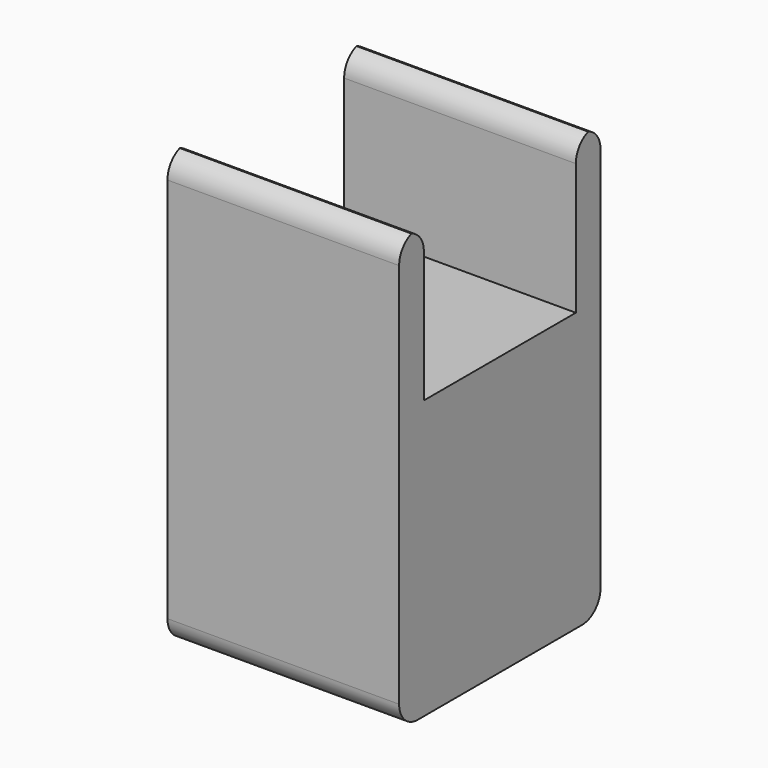
from build123d import *

# Parameters (mm, degrees)
F1_DEPTH    = 7.5
F2_T1_DEPTH = 22.5


# Not quite as in the source:
# - a fillet or chamfer that OpenCascade refuses, or shapes differently, is made with other operations: its cross-section is extruded or revolved along the edge and cut away or added


with BuildPart() as f1:
    # F0 (on Right) → F1 (new body, symmetric)
    with BuildSketch(Plane.YZ):
        Polygon((6.15, 0), (0, 0), (-6.15, 0), (-6.15, 10), (-8.15, 10), (-8.15, -18), (0, -18), (8.15, -18), (8.15, 10), (6.15, 10), align=None)
    extrude(amount=F1_DEPTH, both=True)

    # F2: fillet of radius 1.5 on 6 edges, made by hand

    # F2_s2 → F2_t1 (cut)
    with BuildSketch(Plane.YZ.offset(-11.25)):
        with BuildLine():
            ThreePointArc((-8.15, 8.5), (-7.7106601718, 9.5606601718), (-6.65, 10))
            Line((-6.65, 10), (-8.15, 10))
            Line((-8.15, 10), (-8.15, 8.5))
        make_face()
        with BuildLine():
            ThreePointArc((-7.65, 10), (-6.5893398282, 9.5606601718), (-6.15, 8.5))
            Line((-6.15, 8.5), (-6.15, 10))
            Line((-6.15, 10), (-7.65, 10))
        make_face()
        with BuildLine():
            ThreePointArc((6.15, 8.5), (6.5893398282, 9.5606601718), (7.65, 10))
            Line((7.65, 10), (6.15, 10))
            Line((6.15, 10), (6.15, 8.5))
        make_face()
        with BuildLine():
            ThreePointArc((6.65, 10), (7.7106601718, 9.5606601718), (8.15, 8.5))
            Line((8.15, 8.5), (8.15, 10))
            Line((8.15, 10), (6.65, 10))
        make_face()
        with BuildLine():
            ThreePointArc((-6.65, -18), (-7.7106601718, -17.5606601718), (-8.15, -16.5))
            Line((-8.15, -16.5), (-8.15, -18))
            Line((-8.15, -18), (-6.65, -18))
        make_face()
        with BuildLine():
            ThreePointArc((8.15, -16.5), (7.7106601718, -17.5606601718), (6.65, -18))
            Line((6.65, -18), (8.15, -18))
            Line((8.15, -18), (8.15, -16.5))
        make_face()
    extrude(amount=F2_T1_DEPTH, mode=Mode.SUBTRACT)


solid = f1.part
